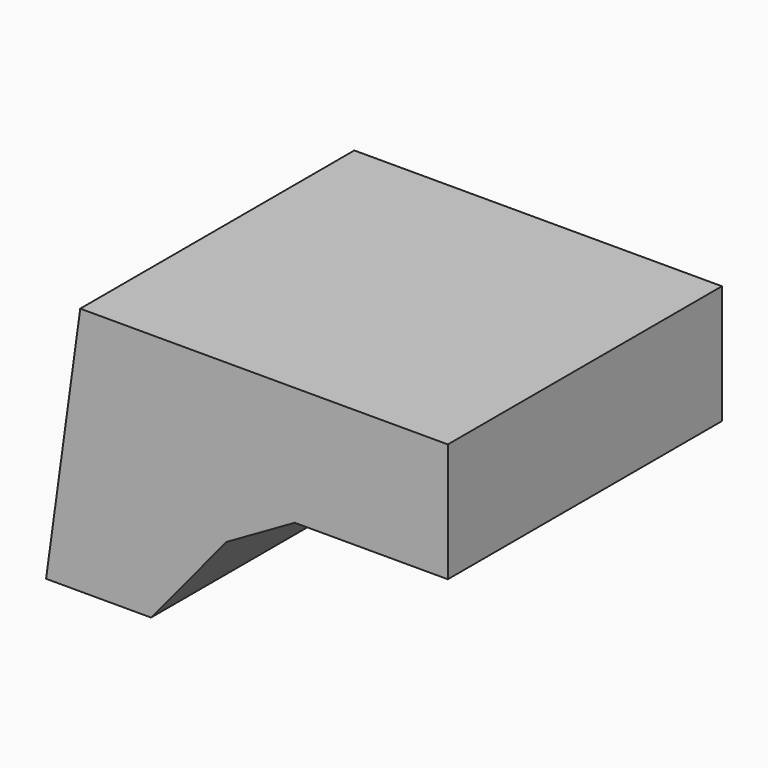
from build123d import *

# Parameters (mm, degrees)
F1_DEPTH = 66.5611065924


# Not quite as in the source:
# - the program builds the solid bodies; features that only make, move or delete a surface that nothing else refers to are left out


with BuildPart() as f1:
    # F0 (on Front) → F1 (new body)
    with BuildSketch(Plane.XZ):
        Polygon((-28.4163840115, 12.6286381856), (-35.0520461798, -35.7411280274), (-14.6560901776, -35.7411280274), (0, -18.0393829942), (13.2530285046, -10.4401372373), (43.007966131, -10.4401372373), (43.007966131, 12.6286381856), (-11.0137574375, 12.6286381856), align=None)
    extrude(amount=-F1_DEPTH)


solid = f1.part
